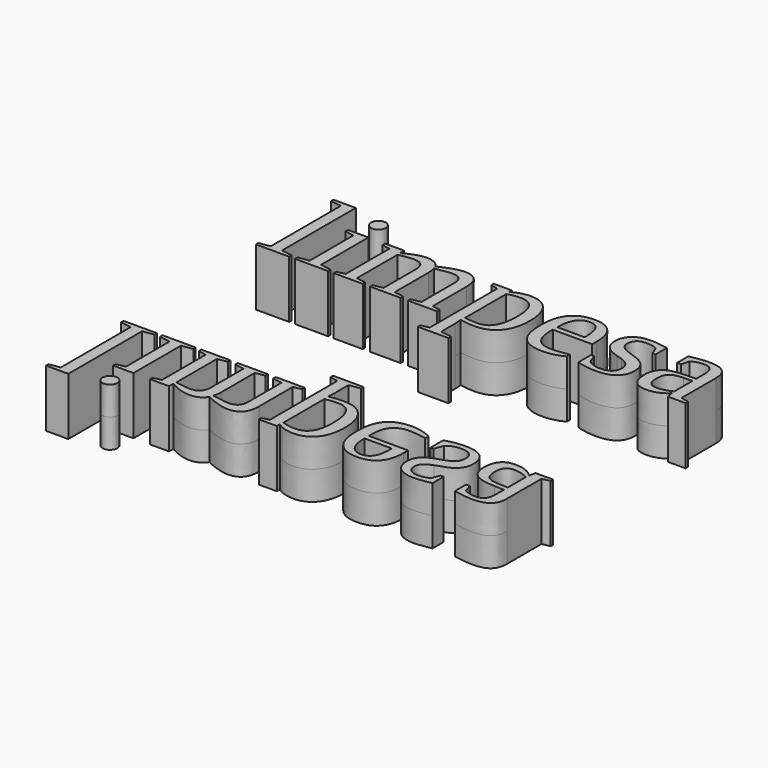
from build123d import *

# Parameters (mm, degrees)
F0_TEXT_SIZE = 121.5147268441
F1_DEPTH     = 25


# Not quite as in the source:
# - Text() gives the source's letters only with a copy of the font that has no kerning and outlines rounded to 1/6400 em; it was checked with that copy


with BuildPart() as f1:
    # F0 (on Top) → F1 (new body, symmetric)
    with BuildSketch(Plane.XY):
        with Locations((-192.2960728407, 72.0282793045)):
            Text('limpesa', F0_TEXT_SIZE, font='Tinos', text_align=(TextAlign.LEFT, TextAlign.BOTTOM))
    extrude(amount=F1_DEPTH, both=True)


with BuildPart() as f2_1:
    # F2: instance of F1
    add(f1.part.mirror(Plane.XZ))


solid = Compound([f1.part, f2_1.part])
